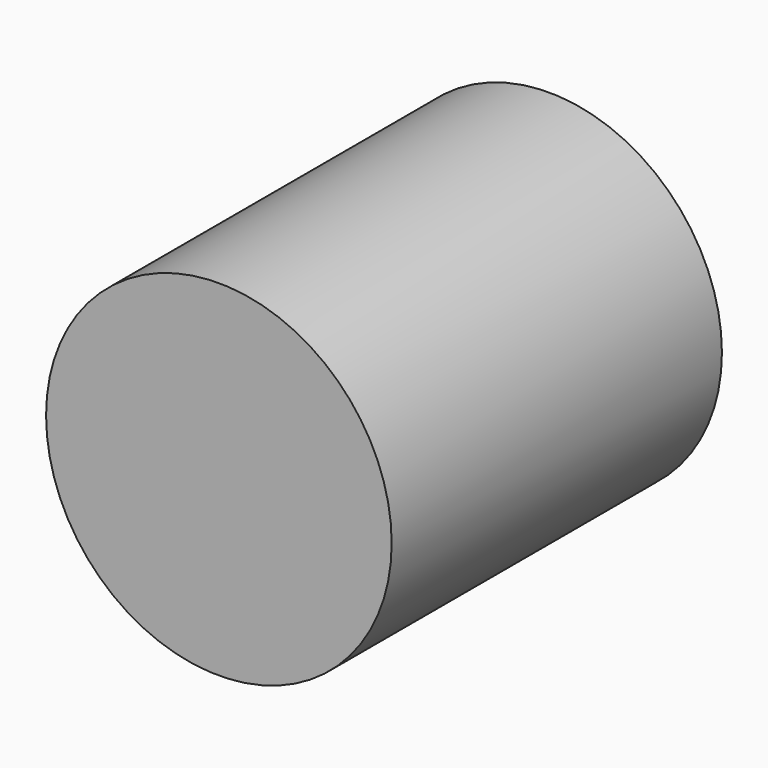
from build123d import *

# Parameters (mm, degrees)
F6_R     = 10.6316838629
F7_DEPTH = 25.4


# Not quite as in the source:
# - a feature of the source that left no trace in its solid (it failed there, or was rolled back) is left out


with BuildPart() as f7:
    # F6 (on Front) → F7 (new body)
    with BuildSketch(Plane.XZ):
        Circle(F6_R)
    extrude(amount=F7_DEPTH)


solid = f7.part
